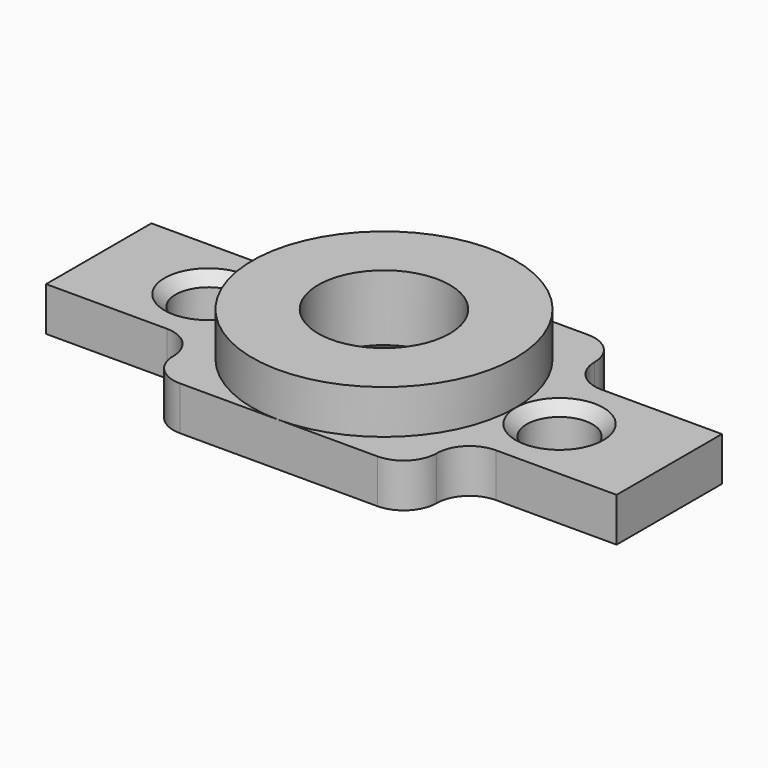
from build123d import *

# Parameters (mm, degrees)
F0_R     = 1.5
F0_R_2   = 3
F1_DEPTH = 2
F2_R     = 6
F2_R_2   = 3
F3_DEPTH = 2
F4_R     = 1.49999
F5_SIZE  = 1
F6_SIZE  = 0.49999


# Not quite as in the source:
# - a fillet or chamfer is up to 0.001 mm smaller than in the source, because OpenCascade refuses the exact size


with BuildPart() as f1:
    # F0 (on Top) → F1 (new body)
    with BuildSketch(Plane.XY):
        Polygon((-6, 3), (-13, 3), (-13, -3), (-6, -3), (-6, -6), (6, -6), (6, -3), (13, -3), (13, 3), (6, 3), (6, 6), (-6, 6), align=None)
        with Locations((-8, 0)):
            Circle(F0_R, mode=Mode.SUBTRACT)
        Circle(F0_R_2, mode=Mode.SUBTRACT)
        with Locations((8, 0)):
            Circle(F0_R, mode=Mode.SUBTRACT)
    extrude(amount=F1_DEPTH)

    # F2 (on face) → F3 (join)
    with BuildSketch(Plane.XY.offset(2)):
        Circle(F2_R)
        Circle(F2_R_2, mode=Mode.SUBTRACT)
    extrude(amount=F3_DEPTH)

    # F4 (radius 1.5 in the source; OpenCascade refuses exactly that, so slightly less here)
    f4_edges = [f1.edges().sort_by_distance(p)[0] for p in [
        (-6, -6, 1),
        (6, -6, 1),
        (6, 6, 1),
        (-6, 6, 1),
        (-6, 3, 1),
        (-6, -3, 1),
        (6, 3, 1),
        (6, -3, 1),
    ]]
    fillet(f4_edges, radius=F4_R)

    # F5
    f5_edges = [f1.edges().sort_by_distance(p)[0] for p in [
        (-3, 0, 0),
    ]]
    chamfer(f5_edges, length=F5_SIZE)

    # F6 (size 0.5 in the source; OpenCascade refuses exactly that, so slightly less here)
    f6_edges = [f1.edges().sort_by_distance(p)[0] for p in [
        (-9.5, 0, 2),
        (6.5, 0, 2),
    ]]
    chamfer(f6_edges, length=F6_SIZE)


solid = f1.part
